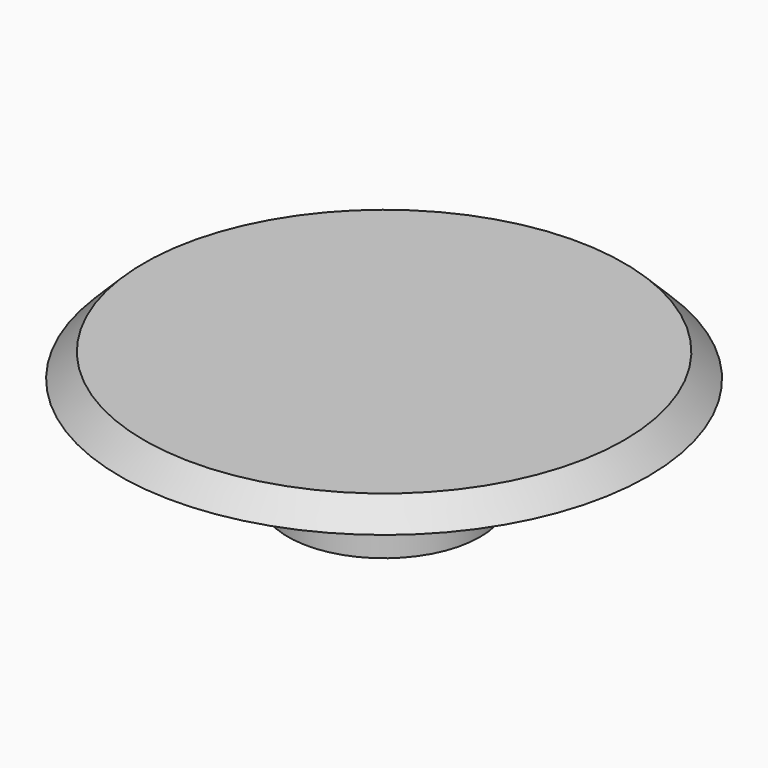
from build123d import *

# Parameters (mm, degrees)
F0_R     = 4
F1_DEPTH = 3.5
F2_R     = 6
F3_DEPTH = 1
F4_R     = 11
F5_DEPTH = 1
F7_SIZE  = 0.99999


# Not quite as in the source:
# - a fillet or chamfer is up to 0.001 mm smaller than in the source, because OpenCascade refuses the exact size


with BuildPart() as f1:
    # F0 (on Top) → F1 (new body)
    with BuildSketch(Plane.XY):
        Circle(F0_R)
    extrude(amount=F1_DEPTH)

    # F2 (on face) → F3 (join)
    with BuildSketch(Plane.XY.offset(3.5)):
        Circle(F2_R)
    extrude(amount=F3_DEPTH)

    # F4 (on face) → F5 (join)
    with BuildSketch(Plane.XY.offset(4.5)):
        Circle(F4_R)
    extrude(amount=F5_DEPTH)

    # F7 (size 1 in the source; OpenCascade refuses exactly that, so slightly less here)
    f7_edges = [f1.edges().sort_by_distance(p)[0] for p in [
        (-11, 0, 5.5),
    ]]
    chamfer(f7_edges, length=F7_SIZE)


solid = f1.part
